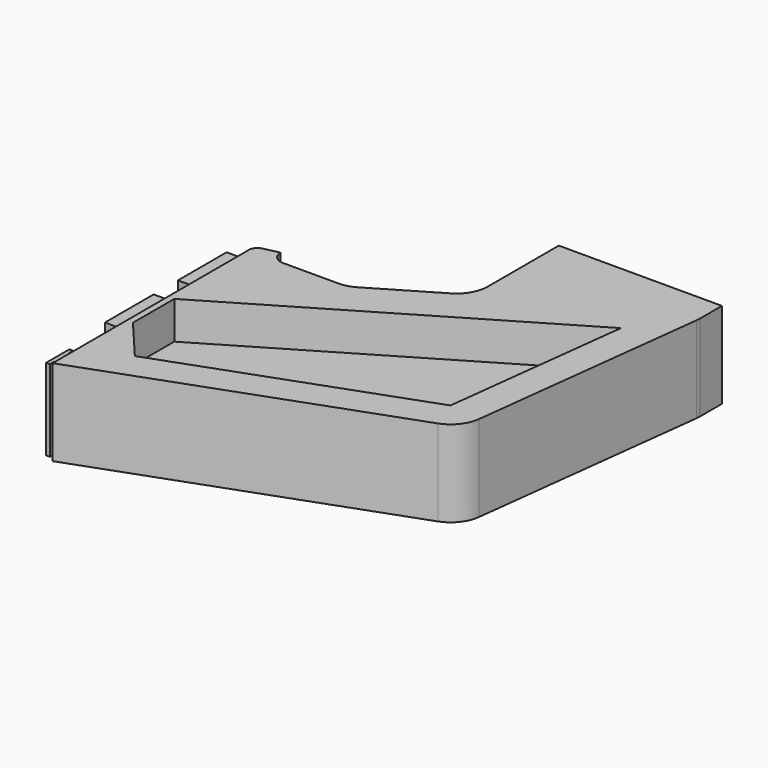
from build123d import *

# Parameters (mm, degrees)
F1_DEPTH = 34.925
F3_DEPTH = 33.02
F4_R     = 12.7
F5_R     = 5.07999
F6_R     = 3.556
F8_DEPTH = 15.24


# Not quite as in the source:
# - a fillet or chamfer is up to 0.001 mm smaller than in the source, because OpenCascade refuses the exact size


with BuildPart() as f1:
    # F0 (on Top) → F1 (new body)
    with BuildSketch(Plane.XY):
        Polygon((9.017, 53.086), (0, 51.054), (0, -51.054), (128.219697074, -4.5338571988), (140.716, 99.822), (140.716, 111.76), (74.676, 111.76), (74.676, 68.58), (39.878, 48.006), (9.017, 48.006), align=None)
    extrude(amount=-F1_DEPTH)

    # F2 (on face) → F3 (join)
    with BuildSketch(Plane(origin=(0, 0, -34.925), x_dir=(1, 0, 0), z_dir=(0, 0, -1))):
        Polygon((-2.0574, -40.767), (0, -40.767), (0, -25.527), (-2.0574, -25.527), (-2.0574, -20.828), (-6.7564, -20.828), (-6.7564, -45.466), (-2.0574, -45.466), align=None)
        Polygon((-2.54, 39.5605), (0, 39.5605), (0, 47.1805), (-2.54, 47.1805), (-2.54, 49.276), (-4.064, 49.276), (-4.064, 37.465), (-2.54, 37.465), align=None)
        Polygon((-2.0574, -3.81), (0, -3.81), (0, 11.43), (-2.0574, 11.43), (-2.0574, 16.129), (-6.7564, 16.129), (-6.7564, -8.509), (-2.0574, -8.509), align=None)
    extrude(amount=-F3_DEPTH)

    # F4
    f4_edges = [f1.edges().sort_by_distance(p)[0] for p in [
        (39.878, 48.006, -17.4625),
        (74.676, 68.58, -17.4625),
        (128.219697, -4.533857, -17.4625),
        (140.716, 99.822, -17.4625),
    ]]
    fillet(f4_edges, radius=F4_R)

    # F5 (radius 5.08 in the source; OpenCascade refuses exactly that, so slightly less here)
    f5_edges = [f1.edges().sort_by_distance(p)[0] for p in [
        (9.017, 48.006, -17.4625),
    ]]
    fillet(f5_edges, radius=F5_R)

    # F6
    f6_edges = [f1.edges().sort_by_distance(p)[0] for p in [
        (0, 51.054, -17.4625),
    ]]
    fillet(f6_edges, radius=F6_R)

    # F7 (on face) → F8 (cut)
    with BuildSketch(Plane.XY):
        Polygon((116.3056778405, 4.923799024), (125.2853724235, 79.9126762258), (2.54, 7.34059472), (2.54, -13.589), (17.272, -31.0071923946), align=None)
    extrude(amount=-F8_DEPTH, mode=Mode.SUBTRACT)


solid = f1.part
